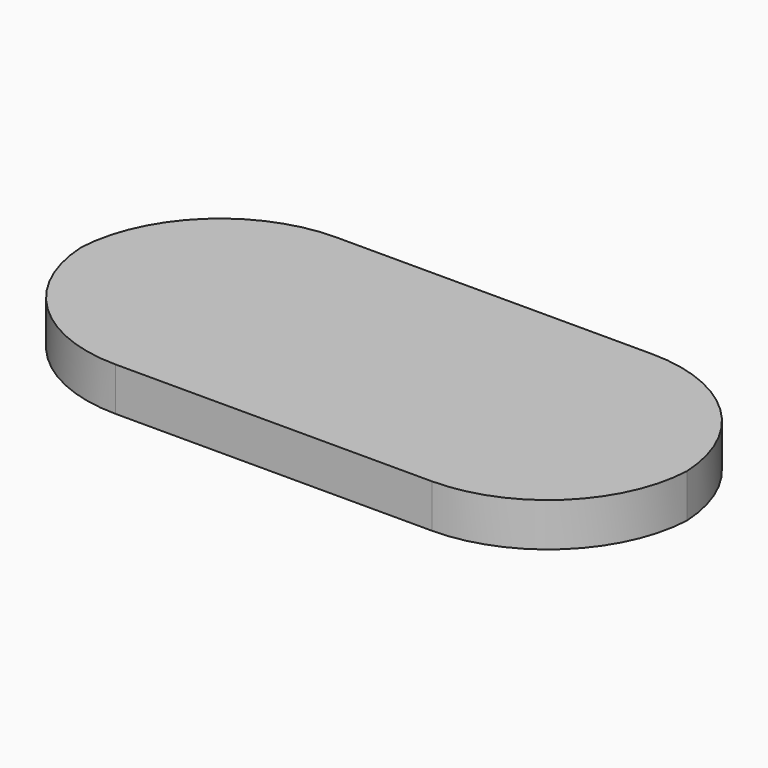
from build123d import *

# Parameters (mm, degrees)
F0_W        = 20.9
F0_H        = 9.5
F1_DEPTH    = 1.5
F2_W        = 16.9
F2_H        = 5.5
F3_DEPTH    = 1
F4_T1_DEPTH = 1
F5_T1_DEPTH = 26.5


# Not quite as in the source:
# - a fillet or chamfer that OpenCascade refuses, or shapes differently, is made with other operations: its cross-section is extruded or revolved along the edge and cut away or added


with BuildPart() as f1:
    # F0 (on Top) → F1 (new body)
    with BuildSketch(Plane.XY):
        with Locations((0.1440625638, -0.617788887)):
            Rectangle(F0_W, F0_H)
    extrude(amount=F1_DEPTH)

    # F2 (on Top) → F3 (cut)
    with BuildSketch(Plane.XY):
        with Locations((0.1440625638, -0.617788887)):
            Rectangle(F2_W, F2_H)
    extrude(amount=F3_DEPTH, mode=Mode.SUBTRACT)

    # F4: fillet of radius 3 on 4 edges, made by hand

    # F4_s2 → F4_t1 (join)
    with BuildSketch(Plane.XY):
        with BuildLine():
            ThreePointArc((8.5940625638, -0.367788887), (7.7153829073, -2.4891092305), (5.5940625638, -3.367788887))
            Line((5.5940625638, -3.367788887), (8.5940625638, -3.367788887))
            Line((8.5940625638, -3.367788887), (8.5940625638, -0.367788887))
        make_face()
        with BuildLine():
            ThreePointArc((-5.3059374362, 2.132211113), (-7.4272577798, 1.2535314566), (-8.3059374362, -0.867788887))
            Line((-8.3059374362, -0.867788887), (-8.3059374362, 2.132211113))
            Line((-8.3059374362, 2.132211113), (-5.3059374362, 2.132211113))
        make_face()
        with BuildLine():
            ThreePointArc((8.5940625638, -0.867788887), (7.7153829073, 1.2535314566), (5.5940625638, 2.132211113))
            Line((5.5940625638, 2.132211113), (8.5940625638, 2.132211113))
            Line((8.5940625638, 2.132211113), (8.5940625638, -0.867788887))
        make_face()
        with BuildLine():
            ThreePointArc((-8.3059374362, -0.367788887), (-7.4272577798, -2.4891092305), (-5.3059374362, -3.367788887))
            Line((-5.3059374362, -3.367788887), (-8.3059374362, -3.367788887))
            Line((-8.3059374362, -3.367788887), (-8.3059374362, -0.367788887))
        make_face()
    extrude(amount=F4_T1_DEPTH)

    # F5: fillet of radius 5 on 4 edges, made by hand

    # F5_s2 → F5_t1 (cut)
    with BuildSketch(Plane.XY.offset(-12.5)):
        with BuildLine():
            ThreePointArc((-10.3059374362, -0.867788887), (-8.8414713422, 2.667745019), (-5.3059374362, 4.132211113))
            Line((-5.3059374362, 4.132211113), (-10.3059374362, 4.132211113))
            Line((-10.3059374362, 4.132211113), (-10.3059374362, -0.867788887))
        make_face()
        with BuildLine():
            ThreePointArc((-5.3059374362, -5.367788887), (-8.8414713422, -3.9033227929), (-10.3059374362, -0.367788887))
            Line((-10.3059374362, -0.367788887), (-10.3059374362, -5.367788887))
            Line((-10.3059374362, -5.367788887), (-5.3059374362, -5.367788887))
        make_face()
        with BuildLine():
            ThreePointArc((10.5940625638, -0.867788887), (9.1295964697, 2.667745019), (5.5940625638, 4.132211113))
            Line((5.5940625638, 4.132211113), (10.5940625638, 4.132211113))
            Line((10.5940625638, 4.132211113), (10.5940625638, -0.867788887))
        make_face()
        with BuildLine():
            ThreePointArc((5.5940625638, -5.367788887), (9.1295964697, -3.9033227929), (10.5940625638, -0.367788887))
            Line((10.5940625638, -0.367788887), (10.5940625638, -5.367788887))
            Line((10.5940625638, -5.367788887), (5.5940625638, -5.367788887))
        make_face()
    extrude(amount=F5_T1_DEPTH, mode=Mode.SUBTRACT)


solid = f1.part
